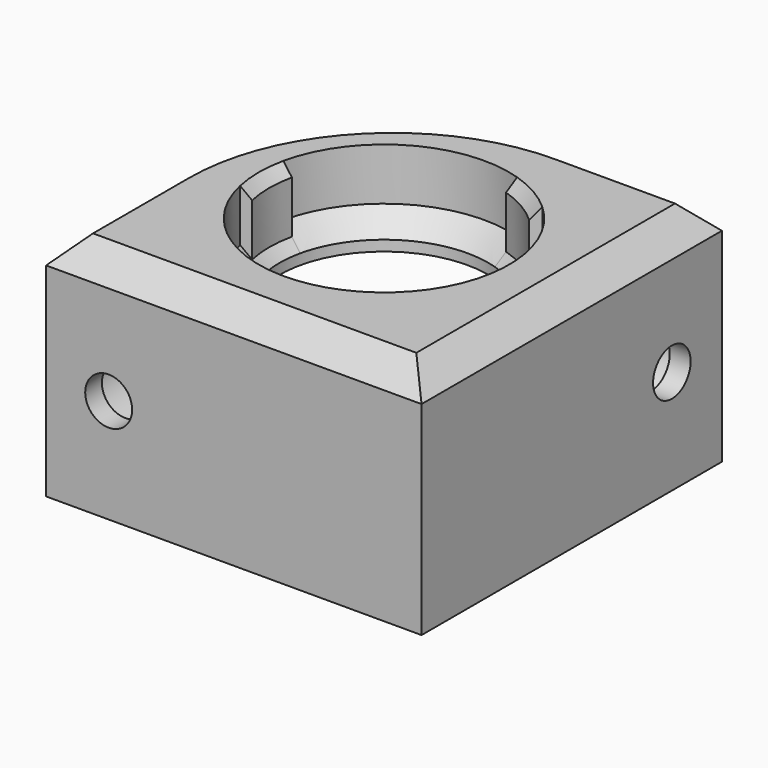
from build123d import *

# Parameters (mm, degrees)
F0_W      = 36
F0_H      = 36
F0_R      = 10
F1_DEPTH  = 8
F3_DEPTH  = 14
F4_R      = 2.25
F5_DEPTH  = 6.001
F6_R      = 3.75
F7_DEPTH  = 4
F8_R      = 2.25
F9_DEPTH  = 6.001
F10_R     = 3.75
F11_DEPTH = 4
F13_DEPTH = 7
F14_R     = 22
F15_SIZE  = 2.5
F16_SIZE  = 0.99999
F17_SIZE  = 1.9999


# Not quite as in the source:
# - a fillet or chamfer is up to 0.001 mm smaller than in the source, because OpenCascade refuses the exact size


with BuildPart() as f1:
    # F0 (on Top) → F1 (new body)
    with BuildSketch(Plane.XY):
        with Locations((18, 18)):
            Rectangle(F0_W, F0_H)
        with Locations((18, 18)):
            Circle(F0_R, mode=Mode.SUBTRACT)
    extrude(amount=F1_DEPTH)

    # F2 (on face) → F3 (join)
    with BuildSketch(Plane(origin=(0, 0, 0), x_dir=(1, 0, 0), z_dir=(0, 0, -1))):
        Polygon((36, 0), (0, 0), (0, -6), (30, -6), (30, -36), (36, -36), align=None)
    extrude(amount=F3_DEPTH)

    # F4 (on face) → F5 (cut, through all)
    with BuildSketch(Plane(origin=(0, 6, 0), x_dir=(-1, 0, 0), z_dir=(0, 1, 0))):
        with Locations((-6, -4)):
            Circle(F4_R)
    extrude(amount=-F5_DEPTH, mode=Mode.SUBTRACT)

    # F6 (on face) → F7 (cut)
    with BuildSketch(Plane(origin=(0, 6, 0), x_dir=(-1, 0, 0), z_dir=(0, 1, 0))):
        with Locations((-6, -4)):
            Circle(F6_R)
    extrude(amount=-F7_DEPTH, mode=Mode.SUBTRACT)

    # F8 (on face) → F9 (cut, through all)
    with BuildSketch(Plane(origin=(30, 0, 0), x_dir=(0, -1, 0), z_dir=(-1, 0, 0))):
        with Locations((-30, -4)):
            Circle(F8_R)
    extrude(amount=-F9_DEPTH, mode=Mode.SUBTRACT)

    # F10 (on face) → F11 (cut)
    with BuildSketch(Plane(origin=(30, 0, 0), x_dir=(0, -1, 0), z_dir=(-1, 0, 0))):
        with Locations((-30, -4)):
            Circle(F10_R)
    extrude(amount=-F11_DEPTH, mode=Mode.SUBTRACT)

    # F12 (on face) → F13 (cut)
    with BuildSketch(Plane.XY.offset(8)):
        with BuildLine():
            Line((21.3077637945, 28.4908864582), (21.6084695941, 29.444603409))
            ThreePointArc((21.6084695941, 29.444603409), (12, 28.3923048454), (6.2844479146, 20.5972753673))
            Line((6.2844479146, 20.5972753673), (7.2607439217, 20.3808357533))
            ThreePointArc((7.2607439217, 20.3808357533), (7, 18), (7.2607439217, 15.6191642467))
            Line((7.2607439217, 15.6191642467), (6.2844479146, 15.4027246327))
            ThreePointArc((6.2844479146, 15.4027246327), (12, 7.6076951546), (21.6084695941, 6.555396591))
            Line((21.6084695941, 6.555396591), (21.3077637945, 7.5091135418))
            ThreePointArc((21.3077637945, 7.5091135418), (23.5, 8.4737205584), (25.4314922838, 9.8899492951))
            Line((25.4314922838, 9.8899492951), (26.1070824914, 9.1526719583))
            ThreePointArc((26.1070824914, 9.1526719583), (30, 18), (26.1070824914, 26.8473280417))
            Line((26.1070824914, 26.8473280417), (25.4314922838, 26.1100507049))
            ThreePointArc((25.4314922838, 26.1100507049), (23.5, 27.5262794416), (21.3077637945, 28.4908864582))
        make_face()
    extrude(amount=-F13_DEPTH, mode=Mode.SUBTRACT)

    # F14
    f14_edges = [f1.edges().sort_by_distance(p)[0] for p in [
        (0, 36, 4),
    ]]
    fillet(f14_edges, radius=F14_R)

    # F15
    f15_edges = [f1.edges().sort_by_distance(p)[0] for p in [
        (36, 18, 8),
        (18, 0, 8),
        (29, 36, 8),
        (0, 7, 8),
    ]]
    chamfer(f15_edges, length=F15_SIZE)

    # F16 (size 1 in the source; OpenCascade refuses exactly that, so slightly less here)
    f16_edges = [f1.edges().sort_by_distance(p)[0] for p in [
        (23.5, 8.473721, 1),
        (7, 18, 1),
        (23.5, 27.526279, 1),
        (7, 18, 8),
        (23.5, 27.526279, 8),
        (23.5, 8.473721, 8),
    ]]
    chamfer(f16_edges, length=F16_SIZE)

    # F17 (size 2 in the source; OpenCascade refuses exactly that, so slightly less here)
    f17_edges = [f1.edges().sort_by_distance(p)[0] for p in [
        (30, 18, 1),
        (12, 7.607695, 1),
        (12, 28.392305, 1),
    ]]
    chamfer(f17_edges, length=F17_SIZE)


solid = f1.part
